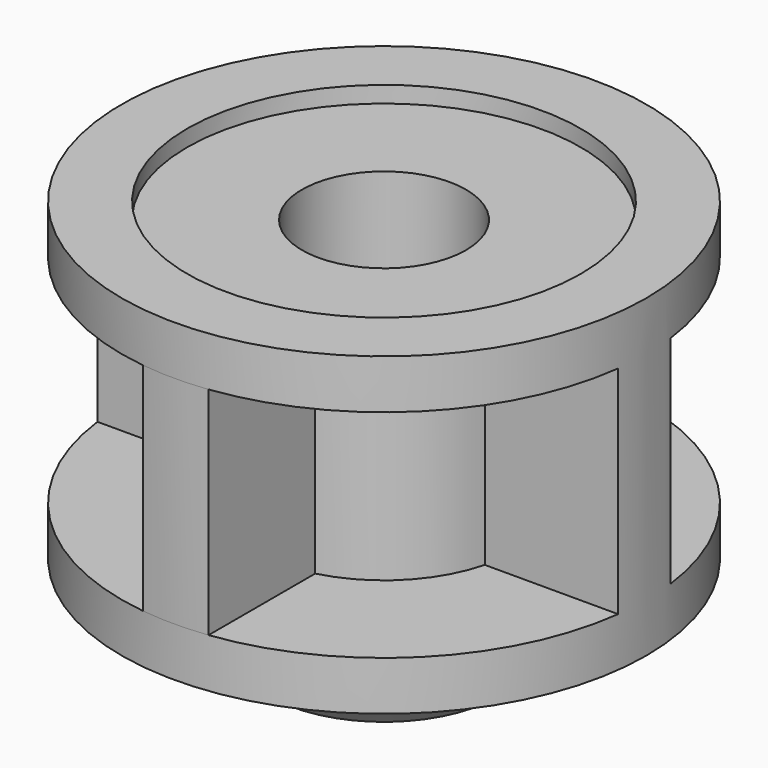
from build123d import *

# Parameters (mm, degrees)
F0_R             = 12.7
F0_R_2           = 3.96875
F1_DEPTH         = 1.5875
F2_R             = 12.7
F2_R_2           = 9.525
F3_DEPTH         = 0.79375
F4_R             = 6.35
F4_R_2           = 3.96875
F5_DEPTH         = 10.4694736
F6_R             = 12.7
F6_R_2           = 3.96875
F7_DEPTH         = 1.5875
F8_R             = 12.7
F8_R_2           = 9.525
F9_DEPTH         = 0.79375
F11_DEPTH        = 10.4694736
F11_COPIES_COUNT = 4
F12_R            = 7.14375
F12_R_2          = 3.96875
F13_DEPTH        = 4.85775
F14_SIZE         = 1.5875


# Not quite as in the source:
# - a length typed as a fraction of an inch, garbled in the dataset ("3 / 203.2 mm" for 3/8 in), is restored
# - a pattern or mirror of a feature is missing from the dataset's text; its kind, count and spacing are read off the source's solid


with BuildPart() as f1:
    # F0 (on Top) → F1 (new body)
    with BuildSketch(Plane.XY):
        Circle(F0_R)
        Circle(F0_R_2, mode=Mode.SUBTRACT)
    extrude(amount=F1_DEPTH)

    # F2 (on face) → F3 (join)
    with BuildSketch(Plane(origin=(0, 0, 0), x_dir=(1, 0, 0), z_dir=(0, 0, -1))):
        Circle(F2_R)
        Circle(F2_R_2, mode=Mode.SUBTRACT)
    extrude(amount=F3_DEPTH)

    # F4 (on face) → F5 (join)
    with BuildSketch(Plane.XY.offset(1.5875)):
        Circle(F4_R)
        Circle(F4_R_2, mode=Mode.SUBTRACT)
    extrude(amount=F5_DEPTH)

    # F6 (on face) → F7 (join)
    with BuildSketch(Plane.XY.offset(12.0569736)):
        Circle(F6_R)
        Circle(F6_R_2, mode=Mode.SUBTRACT)
    extrude(amount=F7_DEPTH)

    # F8 (on face) → F9 (join)
    with BuildSketch(Plane.XY.offset(13.6444736)):
        Circle(F8_R)
        Circle(F8_R_2, mode=Mode.SUBTRACT)
    extrude(amount=F9_DEPTH)

    # F10 (on face) → F11 (join, through all)
    with BuildSketch(Plane.XY.offset(1.5875)):
        with BuildLine():
            Line((1.5875, -12.6003906189), (1.5875, -6.1483610621))
            ThreePointArc((1.5875, -6.1483610621), (0, -6.35), (-1.5875, -6.1483610621))
            Line((-1.5875, -6.1483610621), (-1.5875, -12.6003906189))
            ThreePointArc((-1.5875, -12.6003906189), (0, -12.7), (1.5875, -12.6003906189))
        make_face()
    f11 = extrude(amount=F11_DEPTH)

    # F11_copies: F11 ×4 about axis
    f11_copies_axis = Axis((0, 0, 0), (0, 0, 1))
    for i in range(1, F11_COPIES_COUNT):
        add(f11.rotate(f11_copies_axis, i * 360 / F11_COPIES_COUNT))

    # F12 (on face) → F13 (join)
    with BuildSketch(Plane(origin=(0, 0, 0), x_dir=(1, 0, 0), z_dir=(0, 0, -1))):
        Circle(F12_R)
        Circle(F12_R_2, mode=Mode.SUBTRACT)
    extrude(amount=F13_DEPTH)

    # F14
    f14_edges = [f1.edges().sort_by_distance(p)[0] for p in [
        (-7.14375, 0, -4.85775),
    ]]
    chamfer(f14_edges, length=F14_SIZE)


solid = f1.part
